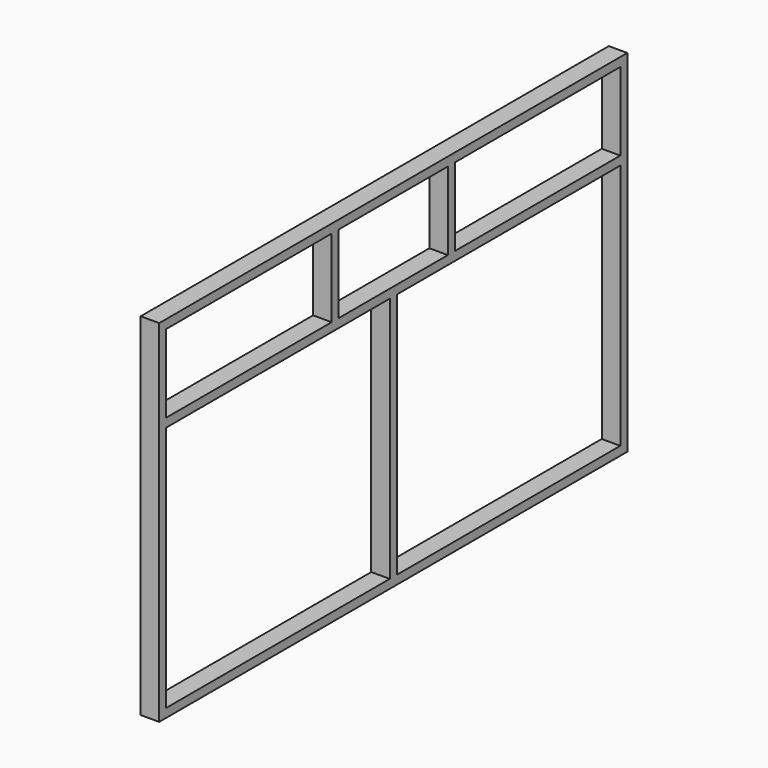
from build123d import *

# Parameters (mm, degrees)
F0_W     = 45
F0_H     = 400
F1_DEPTH = 95


# Not quite as in the source:
# - a feature names something its author has since deleted; it is built from what else it names


with BuildPart() as f1:
    # F0 (on Right) → F1 (new body)
    with BuildSketch(Plane.YZ):
        Polygon((1500, 900), (-1500, 900), (-1500, 855), (-1455, 855), (-395, 855), (-350, 855), (-117.5, 855), (22.5, 855), (350, 855), (395, 855), (1455, 855), (1500, 855), align=None)
        Polygon((-1455, 855), (-1500, 855), (-1500, -855), (-1455, -855), (-1455, 410), (-1455, 455), align=None)
        Polygon((1500, -855), (1500, 855), (1455, 855), (1455, 455), (1455, 410), (1455, 22.5), (1455, -22.5), (1455, -855), align=None)
        Polygon((-1455, -855), (-1500, -855), (-1500, -900), (1500, -900), (1500, -855), (1455, -855), (117.5, -855), (22.5, -855), (-22.5, -855), align=None)
        with Locations((372.5, 655)):
            Rectangle(F0_W, F0_H)
        with Locations((-372.5, 655)):
            Rectangle(F0_W, F0_H)
        Polygon((-395, 455), (-1455, 455), (-1455, 410), (-22.5, 410), (22.5, 410), (1455, 410), (1455, 455), (395, 455), (350, 455), (-350, 455), align=None)
        Polygon((-22.5, 410), (-22.5, -855), (22.5, -855), (22.5, -22.5), (22.5, 22.5), (22.5, 410), align=None)
    extrude(amount=F1_DEPTH)


solid = f1.part
